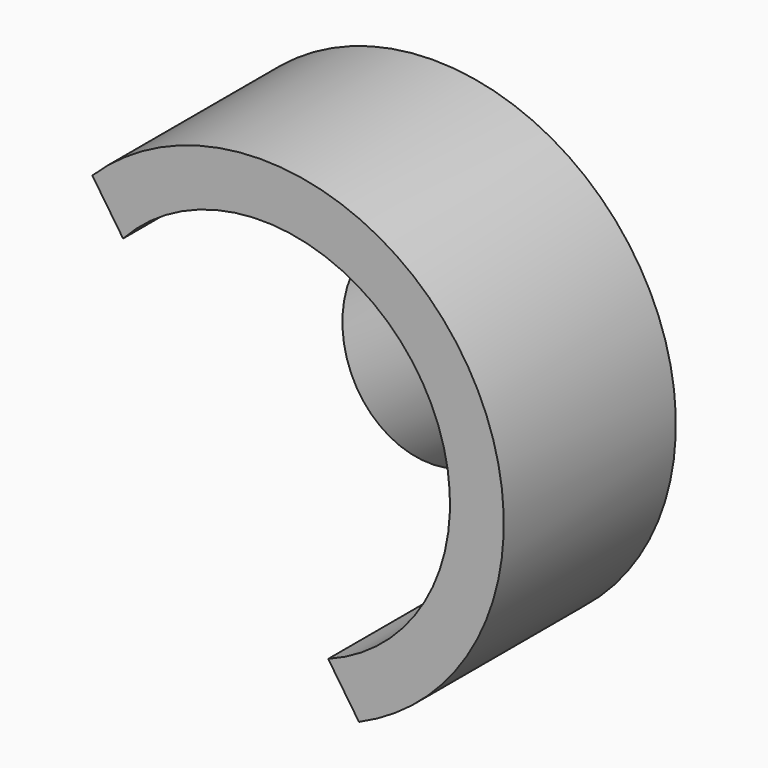
from build123d import *

# Parameters (mm, degrees)
F1_DEPTH = 5.08
F5_R     = 2.286
F6_DEPTH = 2.54


with BuildPart() as f1:
    # F0 (on Front) → F1 (new body)
    with BuildSketch(Plane.XZ):
        with BuildLine():
            ThreePointArc((-3.2760911955, 3.0042056319), (3.6821316631, 2.4899661475), (1.5680416715, -4.1592391512))
            Line((1.5680416715, -4.1592391512), (2.2948386219, -5.2340176442))
            ThreePointArc((2.2948386219, -5.2340176442), (4.7341692811, 3.2013850468), (-4.0028881459, 4.0789841249))
            Line((-4.0028881459, 4.0789841249), (-3.2760911955, 3.0042056319))
        make_face()
    extrude(amount=F1_DEPTH)

    # F5 (on mid) → F6 (join)
    with BuildSketch(Plane(origin=(4.2081504721, 0, 2.8456755972), x_dir=(0, 1, 0), z_dir=(0.8283760772, 0, 0.5601723617))):
        with Locations((-2.54, 0)):
            Circle(F5_R)
    extrude(amount=-F6_DEPTH)


solid = f1.part
